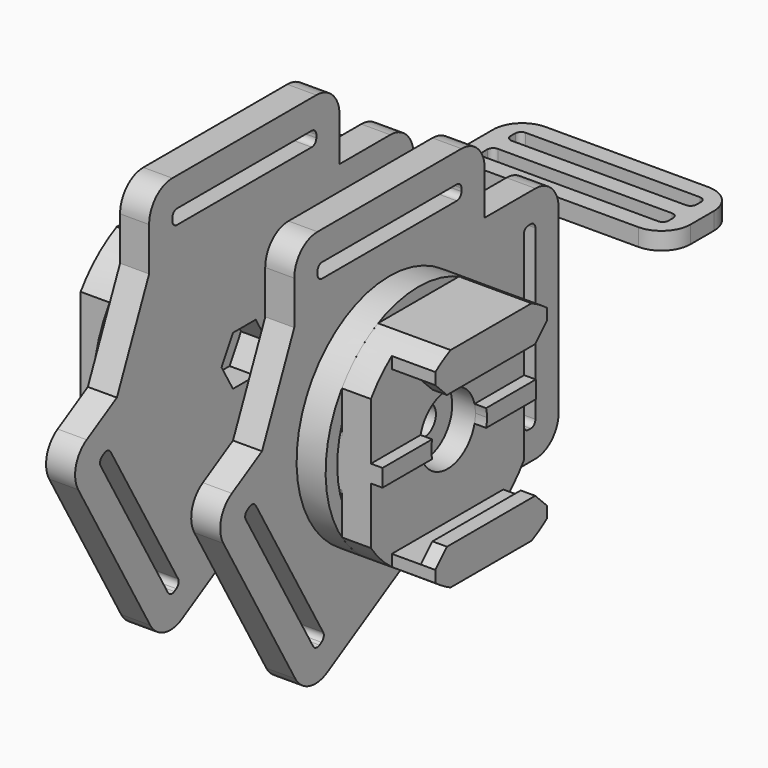
from build123d import *

# Parameters (mm, degrees)
F0_R           = 2.5
F0_W           = 2.5
F0_H           = 31
F0_W_2         = 31
F0_H_2         = 2.5
F1_DEPTH       = 5
F5_DEPTH       = 4.5
F7_DEPTH       = 25
F8_R           = 1
F9_R           = 5
F12_R          = 17
F12_R_2        = 2.5
F13_DEPTH      = 2
F14_W          = 33
F14_H          = 36
F14_R          = 2.5
F15_DEPTH      = 5
F17_DEPTH      = 33
F19_DEPTH      = 7.5
F20_R          = 6
F21_DEPTH      = 4
F21_DEPTH_BACK = 5
F23_DEPTH      = 25
F23_DEPTH_BACK = 25
F24_R          = 17
F24_R_2        = 2.5
F25_DEPTH      = 2
F26_W          = 55
F26_H          = 36
F26_R          = 2.5
F27_DEPTH      = 5
F29_DEPTH      = 33
F31_DEPTH      = 7.5
F32_R          = 4.5
F33_DEPTH      = 5
F33_DEPTH_BACK = 5
F35_DEPTH      = 25
F37_DEPTH      = 7.5
F38_W          = 38
F38_H          = 15
F38_W_2        = 32
F38_H_2        = 3
F39_DEPTH      = 3
F40_R          = 1
F41_R          = 5


with BuildPart() as f1:
    # F0 (on Right) → F1 (new body)
    with BuildSketch(Plane.YZ):
        Polygon((-20.5, 20.5), (-29.5037925243, 20.5), (-29.5037925243, 8.1505087767), (-27.4416511627, 4.5787751659), (-38.26696871, -1.6712248341), (-17.76696871, -37.1782663892), (-6.9416511627, -30.9282663892), (-4.879509801, -34.5), (23.9176880568, -34.5), (23.9176880568, -20.5), (36.4176880568, -20.5), (36.4176880568, 20.5), (23.9176880568, 20.5), (20.5, 20.5), (20.5, 33), (-20.5, 33), align=None)
        Polygon((-15.9368416911, -30.3481393703), (-31.4368416911, -3.501351853), (-29.2717781816, -2.251351853), (-13.7717781816, -29.0981393703), align=None, mode=Mode.SUBTRACT)
        Circle(F0_R, mode=Mode.SUBTRACT)
        with Locations((30.1676880568, 0)):
            Rectangle(F0_W, F0_H, mode=Mode.SUBTRACT)
        with Locations((0, 26.75)):
            Rectangle(F0_W_2, F0_H_2, mode=Mode.SUBTRACT)
    extrude(amount=F1_DEPTH)

    # F2 (on Front) → F3 (revolve)
    with BuildSketch(Plane.XZ):
        Polygon((5, 20), (5, 2.5), (8, 2.5), (8, 17.5), (10, 17.5), (10, 20), align=None)
    revolve(axis=Axis((22.1214631548, 0, 0), (1, 0, 0)))

    # F4 (on face) → F5 (cut)
    with BuildSketch(Plane(origin=(0, 0, 0), x_dir=(0, -1, 0), z_dir=(-1, 0, 0))):
        Polygon((4.9074772881, 0), (2.4537386441, 4.25), (-2.4537386441, 4.25), (-4.9074772881, 0), (-2.4537386441, -4.25), (2.4537386441, -4.25), align=None)
    extrude(amount=-F5_DEPTH, mode=Mode.SUBTRACT)

    # F6 (on face) → F7 (cut)
    with BuildSketch(Plane.YZ.offset(5)):
        Polygon((23.9176880568, -34.5), (23.9176880568, -20.5), (11.1206360583, -20.5), (-6.9416511627, -30.9282663892), (-4.879509801, -34.5), align=None)
        Polygon((-27.4416511627, 4.5787751659), (-20.5, 20.5), (-29.5037925243, 20.5), (-29.5037925243, 8.1505087767), align=None)
    extrude(amount=-F7_DEPTH, mode=Mode.SUBTRACT)

    # F8
    f8_edges = [f1.edges().sort_by_distance(p)[0] for p in [
        (2.5, -15.5, 28),
        (2.5, 15.5, 28),
        (2.5, 15.5, 25.5),
        (2.5, -15.5, 25.5),
        (2.5, 31.417688, 15.5),
        (2.5, 28.917688, 15.5),
        (2.5, 31.417688, -15.5),
        (2.5, 28.917688, -15.5),
        (2.5, -13.771778, -29.098139),
        (2.5, -15.936842, -30.348139),
        (2.5, -29.271778, -2.251352),
        (2.5, -31.436842, -3.501352),
    ]]
    fillet(f8_edges, radius=F8_R)

    # F9
    f9_edges = [f1.edges().sort_by_distance(p)[0] for p in [
        (2.5, -20.5, 33),
        (2.5, 20.5, 33),
        (2.5, 36.417688, 20.5),
        (2.5, 36.417688, -20.5),
        (2.5, -38.266969, -1.671225),
        (2.5, -17.766969, -37.178266),
    ]]
    fillet(f9_edges, radius=F9_R)


with BuildPart() as f11_1:
    # F11: instance of F1
    add(f1.part.mirror(Plane.YZ.offset(-10)))


with BuildPart() as f13:
    # F12 (on face) → F13 (new body)
    with BuildSketch(Plane.YZ.offset(8)):
        Circle(F12_R)
        Circle(F12_R_2, mode=Mode.SUBTRACT)
    extrude(amount=F13_DEPTH)

    # F14 (on face) → F15 (join)
    with BuildSketch(Plane.YZ.offset(10)):
        Rectangle(F14_W, F14_H)
        Circle(F14_R, mode=Mode.SUBTRACT)
    extrude(amount=F15_DEPTH)

    # F16 (on face) → F17 (join, through all)
    with BuildSketch(Plane.XZ.offset(16.5)):
        Polygon((17, -1.5), (17, 0), (17, 1.5), (15, 1.5), (15, 0), (15, -1.5), align=None)
        Polygon((15, 18), (15, 14), (20, 14), (20, 11.5), (22.5, 11.5), (22.5, 18), align=None)
        Polygon((15, -18), (22.5, -18), (22.5, -11.5), (20, -11.5), (20, -14), (15, -14), align=None)
    extrude(amount=-F17_DEPTH)

    # F18 (on face) → F19 (cut, through all)
    with BuildSketch(Plane.YZ.offset(22.5)):
        Polygon((12, 14), (9.5, 11.5), (19.2483495921, 11.5), (19.2483495921, 23.1776126369), (0, 23.1776126369), (-19.2483495921, 23.1776126369), (-19.2483495921, 11.5), (-9.5, 11.5), (-12, 14), (-12, 18), (0, 18), (12, 18), align=None)
        Polygon((-19.2483495921, -11.5), (-19.2483495921, -23.1776126369), (0, -23.1776126369), (19.2483495921, -23.1776126369), (19.2483495921, -11.5), (9.5, -11.5), (12, -14), (12, -18), (0, -18), (-12, -18), (-12, -14), (-9.5, -11.5), align=None)
    extrude(amount=-F19_DEPTH, mode=Mode.SUBTRACT)

    # F20 (on face) → F21 (cut, two sides)
    with BuildSketch(Plane.YZ.offset(15)) as f21_sk:
        Circle(F20_R)
    extrude(amount=-F21_DEPTH, mode=Mode.SUBTRACT)
    extrude(f21_sk.sketch, amount=F21_DEPTH_BACK, mode=Mode.SUBTRACT)

    # F22 (on face) → F23 (cut, two sides)
    with BuildSketch(Plane(origin=(10, 0, 0), x_dir=(0, -1, 0), z_dir=(-1, 0, 0))) as f23_sk:
        Polygon((23.3375262469, 21.4987713844), (0, 21.4987713844), (-23.3375262469, 21.4987713844), (-23.3375262469, -22.0460519195), (0, -22.0460519195), (23.3375262469, -22.0460519195), align=None)
        with BuildLine():
            ThreePointArc((16.5, -11.3026545555), (0, -20), (-16.5, -11.3026545555))
            Line((-16.5, -11.3026545555), (-16.5, 11.3026545555))
            ThreePointArc((-16.5, 11.3026545555), (0, 20), (16.5, 11.3026545555))
            Line((16.5, 11.3026545555), (16.5, -11.3026545555))
        make_face(mode=Mode.SUBTRACT)
    extrude(amount=-F23_DEPTH, mode=Mode.SUBTRACT)
    extrude(f23_sk.sketch, amount=F23_DEPTH_BACK, mode=Mode.SUBTRACT)


with BuildPart() as f25:
    # F24 (on face) → F25 (new body)
    with BuildSketch(Plane(origin=(-28, 0, 0), x_dir=(0, -1, 0), z_dir=(-1, 0, 0))):
        Circle(F24_R)
        Circle(F24_R_2, mode=Mode.SUBTRACT)
    extrude(amount=F25_DEPTH)

    # F26 (on face) → F27 (join)
    with BuildSketch(Plane(origin=(-30, 0, 0), x_dir=(0, -1, 0), z_dir=(-1, 0, 0))):
        with Locations((-11, 0)):
            Rectangle(F26_W, F26_H)
        Circle(F26_R, mode=Mode.SUBTRACT)
    extrude(amount=F27_DEPTH)

    # F28 (on face) → F29 (join)
    with BuildSketch(Plane(origin=(0, 38.5, 0), x_dir=(-1, 0, 0), z_dir=(0, 1, 0))):
        Polygon((37, -1.5), (37, 0), (37, 1.5), (35, 1.5), (35, 0), (35, -1.5), align=None)
        Polygon((35, 18), (35, 14), (40, 14), (40, 11.5), (42.5, 11.5), (42.5, 18), align=None)
        Polygon((35, -14), (35, -18), (42.5, -18), (42.5, -11.5), (40, -11.5), (40, -14), align=None)
    extrude(amount=-F29_DEPTH)

    # F30 (on face) → F31 (cut, through all)
    with BuildSketch(Plane(origin=(-42.5, 0, 0), x_dir=(0, -1, 0), z_dir=(-1, 0, 0))):
        Polygon((-10, 14), (-12.5, 11.5), (-5.5, 11.5), (-5.5, 18), (-10, 18), align=None)
        Polygon((-38.5, 18), (-38.5, 11.5), (-31.5, 11.5), (-34, 14), (-34, 18), align=None)
        Polygon((-5.5, -11.5), (-12.5, -11.5), (-10, -14), (-10, -18), (-5.5, -18), align=None)
        Polygon((-34, -18), (-34, -14), (-31.5, -11.5), (-38.5, -11.5), (-38.5, -18), align=None)
    extrude(amount=-F31_DEPTH, mode=Mode.SUBTRACT)

    # F32 (on face) → F33 (cut, two sides)
    with BuildSketch(Plane(origin=(-35, 0, 0), x_dir=(0, -1, 0), z_dir=(-1, 0, 0))) as f33_sk:
        Circle(F32_R)
    extrude(amount=-F33_DEPTH, mode=Mode.SUBTRACT)
    extrude(f33_sk.sketch, amount=F33_DEPTH_BACK, mode=Mode.SUBTRACT)

    # F34 (on face) → F35 (cut)
    with BuildSketch(Plane(origin=(-42.5, 0, 0), x_dir=(0, -1, 0), z_dir=(-1, 0, 0))):
        with BuildLine():
            ThreePointArc((-30.7177978871, -18), (-35.0459933148, -15.1592235431), (-38.5, -11.3026545555))
            Line((-38.5, -11.3026545555), (-38.5, -18))
            Line((-38.5, -18), (-30.7177978871, -18))
        make_face()
        with BuildLine():
            ThreePointArc((16.5, -11.3026545555), (13.0459933148, -15.1592235431), (8.7177978871, -18))
            Line((8.7177978871, -18), (16.5, -18))
            Line((16.5, -18), (20.9183059633, -18))
            Line((20.9183059633, -18), (20.9183059633, 18))
            Line((20.9183059633, 18), (16.5, 18))
            Line((16.5, 18), (8.7177978871, 18))
            ThreePointArc((8.7177978871, 18), (13.0459933148, 15.1592235431), (16.5, 11.3026545555))
            Line((16.5, 11.3026545555), (16.5, -11.3026545555))
        make_face()
        with BuildLine():
            Line((-30.7177978871, 18), (-38.5, 18))
            Line((-38.5, 18), (-38.5, 11.3026545555))
            ThreePointArc((-38.5, 11.3026545555), (-35.0459933148, 15.1592235431), (-30.7177978871, 18))
        make_face()
    extrude(amount=-F35_DEPTH, mode=Mode.SUBTRACT)

    # F36 (on face) → F37 (cut, through all)
    with BuildSketch(Plane(origin=(-42.5, 0, 0), x_dir=(0, -1, 0), z_dir=(-1, 0, 0))):
        with BuildLine():
            Line((-10, 18), (-13.2822021129, 18))
            ThreePointArc((-13.2822021129, 18), (-11.5929453099, 17.0790284465), (-10, 16))
            Line((-10, 16), (-10, 18))
        make_face()
        with BuildLine():
            Line((-10, -18), (-10, -16))
            ThreePointArc((-10, -16), (-11.5929453099, -17.0790284465), (-13.2822021129, -18))
            Line((-13.2822021129, -18), (-10, -18))
        make_face()
    extrude(amount=-F37_DEPTH, mode=Mode.SUBTRACT)


with BuildPart() as f39:
    # F38 (on Top) → F39 (new body)
    with BuildSketch(Plane.XY):
        with Locations((-12.1502242982, 65.0151353329)):
            Rectangle(F38_W, F38_H)
        with Locations((-12.1502242982, 62.0151353329)):
            Rectangle(F38_W_2, F38_H_2, mode=Mode.SUBTRACT)
        with Locations((-12.1502242982, 68.0151353329)):
            Rectangle(F38_W_2, F38_H_2, mode=Mode.SUBTRACT)
    extrude(amount=F39_DEPTH)

    # F40
    f40_edges = [f39.edges().sort_by_distance(p)[0] for p in [
        (3.849776, 69.515135, 1.5),
        (3.849776, 63.515135, 1.5),
        (-28.150224, 69.515135, 1.5),
        (-28.150224, 63.515135, 1.5),
        (-28.150224, 60.515135, 1.5),
        (-28.150224, 66.515135, 1.5),
        (3.849776, 60.515135, 1.5),
        (3.849776, 66.515135, 1.5),
    ]]
    fillet(f40_edges, radius=F40_R)

    # F41
    f41_edges = [f39.edges().sort_by_distance(p)[0] for p in [
        (6.849776, 57.515135, 1.5),
        (6.849776, 72.515135, 1.5),
        (-31.150224, 57.515135, 1.5),
        (-31.150224, 72.515135, 1.5),
    ]]
    fillet(f41_edges, radius=F41_R)


solid = Compound([f1.part, f11_1.part, f13.part, f25.part, f39.part])
